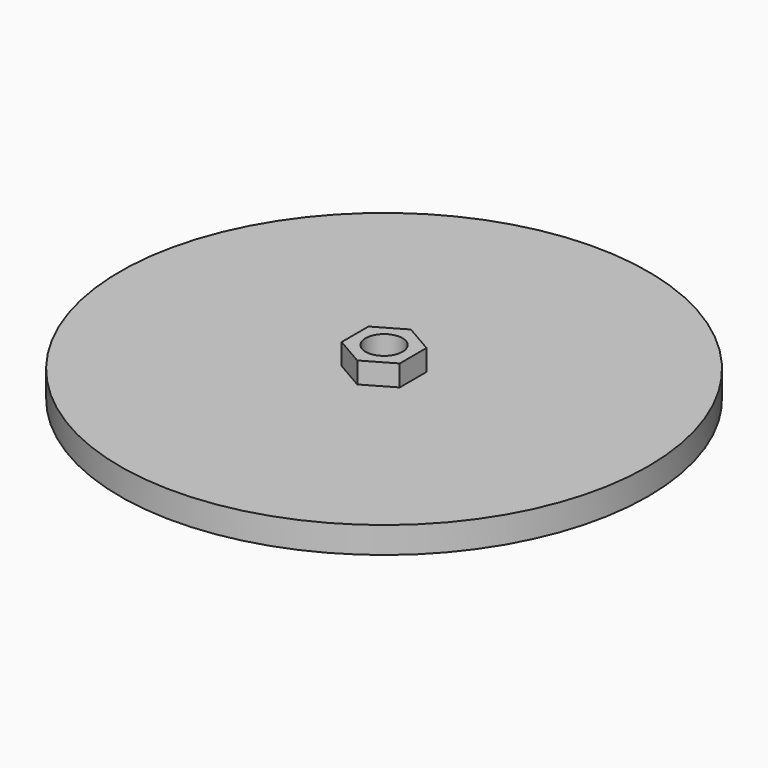
from build123d import *

# Parameters (mm, degrees)
F0_R     = 27.5
F1_DEPTH = 6
F2_R     = 7
F3_DEPTH = 30
F4_R     = 7
F5_DEPTH = 8
F6_R     = 100
F6_R_2   = 7
F7_DEPTH = 10


with BuildPart() as f1:
    # F0 (on Top) → F1 (new body)
    with BuildSketch(Plane.XY):
        Circle(F0_R)
    extrude(amount=F1_DEPTH)

    # F2 (on face) → F3 (join)
    with BuildSketch(Plane.XY):
        Circle(F2_R)
    extrude(amount=-F3_DEPTH)


with BuildPart() as f5:
    # F4 (on face) → F5 (new body)
    with BuildSketch(Plane(origin=(0, 0, -30), x_dir=(1, 0, 0), z_dir=(0, 0, -1))):
        Polygon((11, -6.3508529611), (11, 6.3508529611), (0, 12.7017059222), (-11, 6.3508529611), (-11, -6.3508529611), (0, -12.7017059222), align=None)
        Circle(F4_R, mode=Mode.SUBTRACT)
    extrude(amount=F5_DEPTH)


with BuildPart() as f7:
    # F6 (on face) → F7 (new body)
    with BuildSketch(Plane(origin=(0, 0, -38), x_dir=(1, 0, 0), z_dir=(0, 0, -1))):
        Circle(F6_R)
        Polygon((11, -6.3508529611), (0, -12.7017059222), (-11, -6.3508529611), (-11, 6.3508529611), (0, 12.7017059222), (11, 6.3508529611), align=None, mode=Mode.SUBTRACT)
        Polygon((-11, -6.3508529611), (0, -12.7017059222), (11, -6.3508529611), (11, 6.3508529611), (0, 12.7017059222), (-11, 6.3508529611), align=None)
        Circle(F6_R_2, mode=Mode.SUBTRACT)
        Circle(F6_R_2)
    extrude(amount=F7_DEPTH)


solid = Compound([f5.part, f7.part])
